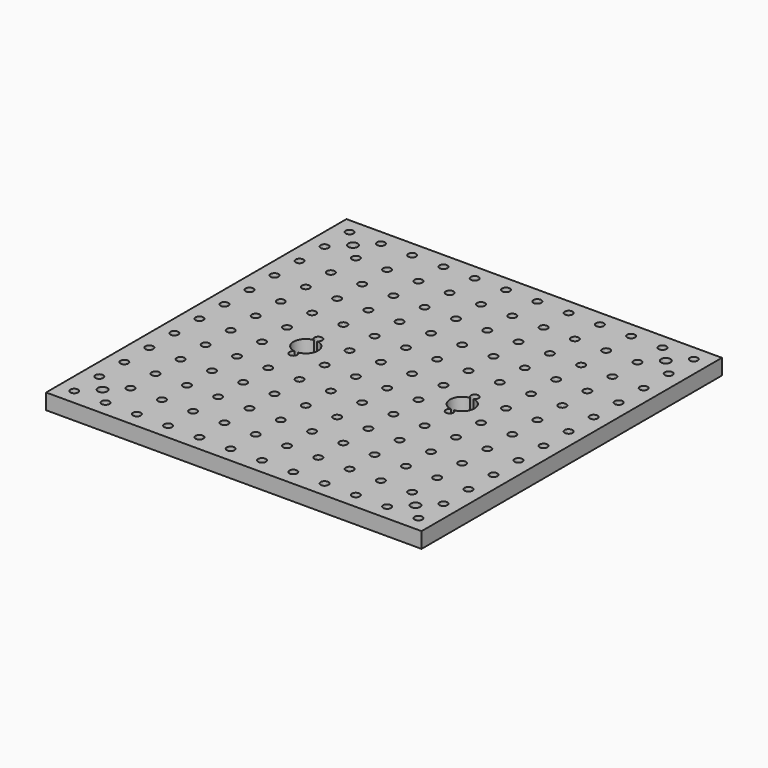
from build123d import *

# Parameters (mm, degrees)
F0_W     = 304.8
F0_H     = 304.8
F1_DEPTH = 12.7
F2_R     = 3.175
F2_R_2   = 3.81
F3_DEPTH = 25.4
F4_R     = 9.92124
F5_DEPTH = 25.4


# Not quite as in the source:
# - a pattern or mirror of a feature is missing from the dataset's text; its kind, count and spacing are read off the source's solid


with BuildPart() as f1:
    # F0 (on Top) → F1 (new body)
    with BuildSketch(Plane.XY):
        Rectangle(F0_W, F0_H)
    extrude(amount=F1_DEPTH)

    # F2 (on face) → F3 (cut)
    with BuildSketch(Plane.XY.offset(12.7)):
        with Locations((-139.7, -139.7)):
            Circle(F2_R)
        with Locations((-139.7, -114.3)):
            Circle(F2_R)
        with Locations((-139.7, -88.9)):
            Circle(F2_R)
        with Locations((-139.7, -63.5)):
            Circle(F2_R)
        with Locations((-139.7, -38.1)):
            Circle(F2_R)
        with Locations((-139.7, -12.7)):
            Circle(F2_R)
        with Locations((-139.7, 12.7)):
            Circle(F2_R)
        with Locations((-139.7, 38.1)):
            Circle(F2_R)
        with Locations((-139.7, 63.5)):
            Circle(F2_R)
        with Locations((-139.7, 88.9)):
            Circle(F2_R)
        with Locations((-139.7, 114.3)):
            Circle(F2_R)
        with Locations((-114.3, -139.7)):
            Circle(F2_R)
        with Locations((-114.3, -114.3)):
            Circle(F2_R)
        with Locations((-114.3, -88.9)):
            Circle(F2_R)
        with Locations((-114.3, -63.5)):
            Circle(F2_R)
        with Locations((-114.3, -38.1)):
            Circle(F2_R)
        with Locations((-114.3, -12.7)):
            Circle(F2_R)
        with Locations((-114.3, 12.7)):
            Circle(F2_R)
        with Locations((-114.3, 38.1)):
            Circle(F2_R)
        with Locations((-114.3, 63.5)):
            Circle(F2_R)
        with Locations((-114.3, 88.9)):
            Circle(F2_R)
        with Locations((-114.3, 114.3)):
            Circle(F2_R)
        with Locations((-88.9, -139.7)):
            Circle(F2_R)
        with Locations((-88.9, -114.3)):
            Circle(F2_R)
        with Locations((-88.9, -88.9)):
            Circle(F2_R)
        with Locations((-88.9, -63.5)):
            Circle(F2_R)
        with Locations((-88.9, -38.1)):
            Circle(F2_R)
        with Locations((-88.9, -12.7)):
            Circle(F2_R)
        with Locations((-88.9, 12.7)):
            Circle(F2_R)
        with Locations((-88.9, 38.1)):
            Circle(F2_R)
        with Locations((-88.9, 63.5)):
            Circle(F2_R)
        with Locations((-88.9, 88.9)):
            Circle(F2_R)
        with Locations((-88.9, 114.3)):
            Circle(F2_R)
        with Locations((-63.5, -139.7)):
            Circle(F2_R)
        with Locations((-63.5, -114.3)):
            Circle(F2_R)
        with Locations((-63.5, -88.9)):
            Circle(F2_R)
        with Locations((-63.5, -63.5)):
            Circle(F2_R)
        with Locations((-63.5, -38.1)):
            Circle(F2_R)
        with Locations((-63.5, -12.7)):
            Circle(F2_R)
        with Locations((-63.5, 12.7)):
            Circle(F2_R)
        with Locations((-63.5, 38.1)):
            Circle(F2_R)
        with Locations((-63.5, 63.5)):
            Circle(F2_R)
        with Locations((-63.5, 88.9)):
            Circle(F2_R)
        with Locations((-63.5, 114.3)):
            Circle(F2_R)
        with Locations((-38.1, -139.7)):
            Circle(F2_R)
        with Locations((-38.1, -114.3)):
            Circle(F2_R)
        with Locations((-38.1, -88.9)):
            Circle(F2_R)
        with Locations((-38.1, -63.5)):
            Circle(F2_R)
        with Locations((-38.1, -38.1)):
            Circle(F2_R)
        with Locations((-38.1, -12.7)):
            Circle(F2_R)
        with Locations((-38.1, 12.7)):
            Circle(F2_R)
        with Locations((-38.1, 38.1)):
            Circle(F2_R)
        with Locations((-38.1, 63.5)):
            Circle(F2_R)
        with Locations((-38.1, 88.9)):
            Circle(F2_R)
        with Locations((-38.1, 114.3)):
            Circle(F2_R)
        with Locations((-12.7, -139.7)):
            Circle(F2_R)
        with Locations((-12.7, -114.3)):
            Circle(F2_R)
        with Locations((-12.7, -88.9)):
            Circle(F2_R)
        with Locations((-12.7, -63.5)):
            Circle(F2_R)
        with Locations((-12.7, -38.1)):
            Circle(F2_R)
        with Locations((-12.7, -12.7)):
            Circle(F2_R)
        with Locations((-12.7, 12.7)):
            Circle(F2_R)
        with Locations((-12.7, 38.1)):
            Circle(F2_R)
        with Locations((-12.7, 63.5)):
            Circle(F2_R)
        with Locations((-12.7, 88.9)):
            Circle(F2_R)
        with Locations((-12.7, 114.3)):
            Circle(F2_R)
        with Locations((12.7, -139.7)):
            Circle(F2_R)
        with Locations((12.7, -114.3)):
            Circle(F2_R)
        with Locations((12.7, -88.9)):
            Circle(F2_R)
        with Locations((12.7, -63.5)):
            Circle(F2_R)
        with Locations((12.7, -38.1)):
            Circle(F2_R)
        with Locations((12.7, -12.7)):
            Circle(F2_R)
        with Locations((12.7, 12.7)):
            Circle(F2_R)
        with Locations((12.7, 38.1)):
            Circle(F2_R)
        with Locations((12.7, 63.5)):
            Circle(F2_R)
        with Locations((12.7, 88.9)):
            Circle(F2_R)
        with Locations((12.7, 114.3)):
            Circle(F2_R)
        with Locations((38.1, -139.7)):
            Circle(F2_R)
        with Locations((38.1, -114.3)):
            Circle(F2_R)
        with Locations((38.1, -88.9)):
            Circle(F2_R)
        with Locations((38.1, -63.5)):
            Circle(F2_R)
        with Locations((38.1, -38.1)):
            Circle(F2_R)
        with Locations((38.1, -12.7)):
            Circle(F2_R)
        with Locations((38.1, 12.7)):
            Circle(F2_R)
        with Locations((38.1, 38.1)):
            Circle(F2_R)
        with Locations((38.1, 63.5)):
            Circle(F2_R)
        with Locations((38.1, 88.9)):
            Circle(F2_R)
        with Locations((38.1, 114.3)):
            Circle(F2_R)
        with Locations((63.5, -139.7)):
            Circle(F2_R)
        with Locations((63.5, -114.3)):
            Circle(F2_R)
        with Locations((63.5, -88.9)):
            Circle(F2_R)
        with Locations((63.5, -63.5)):
            Circle(F2_R)
        with Locations((63.5, -38.1)):
            Circle(F2_R)
        with Locations((63.5, -12.7)):
            Circle(F2_R)
        with Locations((63.5, 12.7)):
            Circle(F2_R)
        with Locations((63.5, 38.1)):
            Circle(F2_R)
        with Locations((63.5, 63.5)):
            Circle(F2_R)
        with Locations((63.5, 88.9)):
            Circle(F2_R)
        with Locations((63.5, 114.3)):
            Circle(F2_R)
        with Locations((88.9, -139.7)):
            Circle(F2_R)
        with Locations((88.9, -114.3)):
            Circle(F2_R)
        with Locations((88.9, -88.9)):
            Circle(F2_R)
        with Locations((88.9, -63.5)):
            Circle(F2_R)
        with Locations((88.9, -38.1)):
            Circle(F2_R)
        with Locations((88.9, -12.7)):
            Circle(F2_R)
        with Locations((88.9, 12.7)):
            Circle(F2_R)
        with Locations((88.9, 38.1)):
            Circle(F2_R)
        with Locations((88.9, 63.5)):
            Circle(F2_R)
        with Locations((88.9, 88.9)):
            Circle(F2_R)
        with Locations((88.9, 114.3)):
            Circle(F2_R)
        with Locations((114.3, -139.7)):
            Circle(F2_R)
        with Locations((114.3, -114.3)):
            Circle(F2_R)
        with Locations((114.3, -88.9)):
            Circle(F2_R)
        with Locations((114.3, -63.5)):
            Circle(F2_R)
        with Locations((114.3, -38.1)):
            Circle(F2_R)
        with Locations((114.3, -12.7)):
            Circle(F2_R)
        with Locations((114.3, 12.7)):
            Circle(F2_R)
        with Locations((114.3, 38.1)):
            Circle(F2_R)
        with Locations((114.3, 63.5)):
            Circle(F2_R)
        with Locations((114.3, 88.9)):
            Circle(F2_R)
        with Locations((114.3, 114.3)):
            Circle(F2_R)
        with Locations((139.7, -139.7)):
            Circle(F2_R)
        with Locations((139.7, -114.3)):
            Circle(F2_R)
        with Locations((139.7, -88.9)):
            Circle(F2_R)
        with Locations((139.7, -63.5)):
            Circle(F2_R)
        with Locations((139.7, -38.1)):
            Circle(F2_R)
        with Locations((139.7, -12.7)):
            Circle(F2_R)
        with Locations((139.7, 12.7)):
            Circle(F2_R)
        with Locations((139.7, 38.1)):
            Circle(F2_R)
        with Locations((139.7, 63.5)):
            Circle(F2_R)
        with Locations((139.7, 88.9)):
            Circle(F2_R)
        with Locations((139.7, 114.3)):
            Circle(F2_R)
        with Locations((-139.7, 139.7)):
            Circle(F2_R)
        with Locations((-114.3, 139.7)):
            Circle(F2_R)
        with Locations((-88.9, 139.7)):
            Circle(F2_R)
        with Locations((-63.5, 139.7)):
            Circle(F2_R)
        with Locations((-38.1, 139.7)):
            Circle(F2_R)
        with Locations((-12.7, 139.7)):
            Circle(F2_R)
        with Locations((12.7, 139.7)):
            Circle(F2_R)
        with Locations((38.1, 139.7)):
            Circle(F2_R)
        with Locations((63.5, 139.7)):
            Circle(F2_R)
        with Locations((88.9, 139.7)):
            Circle(F2_R)
        with Locations((114.3, 139.7)):
            Circle(F2_R)
        with Locations((139.7, 139.7)):
            Circle(F2_R)
        with Locations((-126.8168389797, -127)):
            Circle(F2_R_2)
        with Locations((-126.8168389797, 127)):
            Circle(F2_R_2)
        with Locations((127.1831610203, -127)):
            Circle(F2_R_2)
        with Locations((127.1831610203, 127)):
            Circle(F2_R_2)
        with Locations((381.1831610203, -127)):
            Circle(F2_R_2)
        with Locations((381.1831610203, 127)):
            Circle(F2_R_2)
    extrude(amount=-F3_DEPTH, mode=Mode.SUBTRACT)

    # F4 (on Top) → F5 (cut)
    with BuildSketch(Plane.XY):
        with Locations((-63.5, 0)):
            Circle(F4_R)
    f5 = extrude(amount=F5_DEPTH, mode=Mode.SUBTRACT)

    # F5_copies: F5 across plane
    add(f5.mirror(Plane(origin=(0, 0, 0), x_dir=(0, 0, 1), z_dir=(1, 0, 0))), mode=Mode.SUBTRACT)


solid = f1.part
